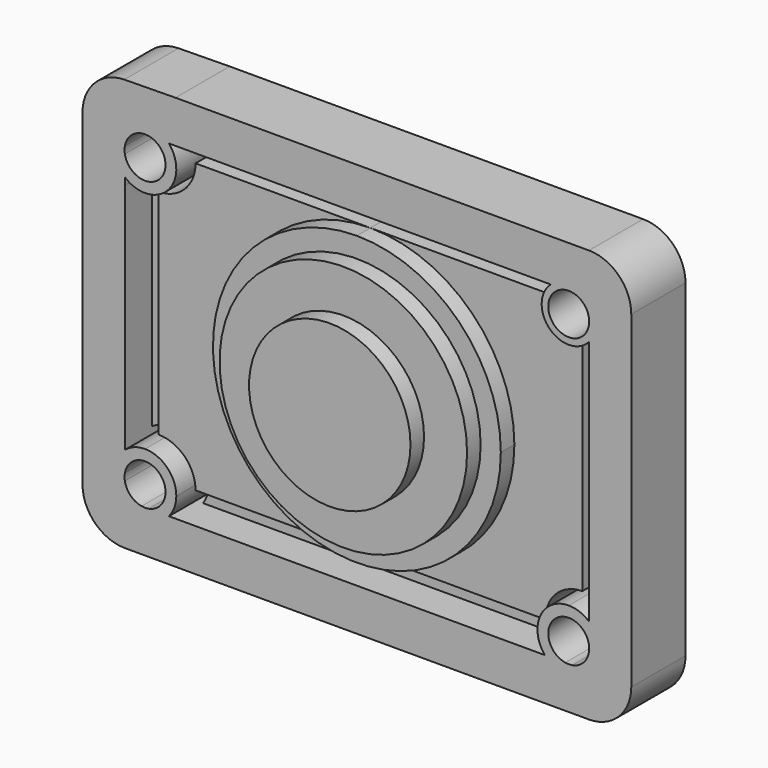
from build123d import *

# Parameters (mm, degrees)
F0_R     = 9.525
F1_DEPTH = 12
F3_DEPTH = 6
F0_R_2   = 14.605
F4_DEPTH = 8
F5_DEPTH = 10
F6_DEPTH = 8
F7_DEPTH = 4


# Not quite as in the source:
# - a feature of the source that left no trace in its solid (it failed there, or was rolled back) is left out


with BuildPart() as f1:
    # F0 (on Front) → F1 (new body)
    with BuildSketch(Plane.XZ):
        with Locations((25, 0.5246010458)):
            Circle(F0_R)
    extrude(amount=F1_DEPTH)


with BuildPart() as f3:
    # F0 (on Front) → F3 (new body)
    with BuildSketch(Plane.XZ):
        with BuildLine():
            ThreePointArc((25, -16.4603989542), (8.015, 0.5246010458), (25, 17.5096010458))
            Line((25, 17.5096010458), (6.92, 17.5096010458))
            Line((6.92, 17.5096010458), (4.365, 17.5096010458))
            ThreePointArc((4.365, 17.5096010458), (3.0865210999, 14.423079946), (0, 13.1446010458))
            Line((0, 13.1446010458), (0, 10.59))
            Line((0, 10.59), (0, 0))
            Line((0, 0), (0, -10.59))
            Line((0, -10.59), (0, -12.0953989542))
            ThreePointArc((0, -12.0953989542), (3.0865210999, -13.3738778543), (4.365, -16.4603989542))
            Line((4.365, -16.4603989542), (25, -16.4603989542))
        make_face()
    extrude(amount=F3_DEPTH)


with BuildPart() as f3b:
    # F0 (on Front) → F3, piece 2 (new body)
    with BuildSketch(Plane.XZ):
        with BuildLine():
            ThreePointArc((25, 17.5096010458), (37.0102086785, 12.5348097243), (41.985, 0.5246010458))
            ThreePointArc((41.985, 0.5246010458), (37.0102086785, -11.4856076326), (25, -16.4603989542))
            Line((25, -16.4603989542), (45.635, -16.4603989542))
            ThreePointArc((45.635, -16.4603989542), (46.9134789001, -13.3738778543), (50, -12.0953989542))
            Line((50, -12.0953989542), (50, 13.8196010458))
            ThreePointArc((50, 13.8196010458), (47.3907759774, 14.9003770233), (46.31, 17.5096010458))
            Line((46.31, 17.5096010458), (25, 17.5096010458))
        make_face()
    extrude(amount=F3_DEPTH)


with BuildPart() as f4:
    # F0 (on Front) → F4 (new body)
    with BuildSketch(Plane.XZ):
        with BuildLine():
            ThreePointArc((25, -16.4603989542), (37.0102086785, -11.4856076326), (41.985, 0.5246010458))
            ThreePointArc((41.985, 0.5246010458), (37.0102086785, 12.5348097243), (25, 17.5096010458))
            ThreePointArc((25, 17.5096010458), (8.015, 0.5246010458), (25, -16.4603989542))
        make_face()
        with Locations((25, 0.5246010458)):
            Circle(F0_R_2, mode=Mode.SUBTRACT)
    extrude(amount=F4_DEPTH)


with BuildPart() as f5:
    # F0 (on Front) → F5 (new body)
    with BuildSketch(Plane.XZ):
        with Locations((25, 0.5246010458)):
            Circle(F0_R_2)
        with Locations((25, 0.5246010458)):
            Circle(F0_R, mode=Mode.SUBTRACT)
    extrude(amount=F5_DEPTH)


with BuildPart() as f6:
    # F0 (on Front) → F6 (new body)
    with BuildSketch(Plane.XZ):
        with BuildLine():
            Line((-7.38, 19.8103227064), (-7.38, 0))
            Line((-7.38, 0), (-7.38, -18.8403989542))
            ThreePointArc((-7.38, -18.8403989542), (-5.9155339059, -22.3759328601), (-2.38, -23.8403989542))
            Line((-2.38, -23.8403989542), (52.38, -23.8403989542))
            ThreePointArc((52.38, -23.8403989542), (55.9155339059, -22.3759328601), (57.38, -18.8403989542))
            Line((57.38, -18.8403989542), (57.38, 0))
            Line((57.38, 0), (57.38, 19.8891702691))
            ThreePointArc((57.38, 19.8891702691), (55.9155339059, 23.4247041751), (52.38, 24.8891702691))
            Line((52.38, 24.8891702691), (3.5934421678, 24.8891702691))
            Line((3.5934421678, 24.8891702691), (-2.4456321687, 24.8098919297))
            ThreePointArc((-2.4456321687, 24.8098919297), (-5.9386627294, 23.3225754847), (-7.38, 19.8103227064))
        make_face()
        with BuildLine():
            ThreePointArc((-0.4096644969, -18.8403989542), (-1.7076628766, -18.1680618307), (-2.38, -16.870063451))
            ThreePointArc((-2.38, -16.870063451), (-2.415, -16.4603989542), (-2.38, -16.0507344573))
            ThreePointArc((-2.38, -16.0507344573), (0.2055784522, -14.0541648633), (2.415, -16.4603989542))
            ThreePointArc((2.415, -16.4603989542), (1.8468303604, -18.0164974793), (0.4096644969, -18.8403989542))
            ThreePointArc((0.4096644969, -18.8403989542), (0, -18.8753989542), (-0.4096644969, -18.8403989542))
        make_face(mode=Mode.SUBTRACT)
        with BuildLine():
            ThreePointArc((52.415, -16.4603989542), (52.4062340909, -16.6659774063), (52.38, -16.870063451))
            ThreePointArc((52.38, -16.870063451), (51.7076628766, -18.1680618307), (50.4096644969, -18.8403989542))
            ThreePointArc((50.4096644969, -18.8403989542), (50, -18.8753989542), (49.5903355031, -18.8403989542))
            ThreePointArc((49.5903355031, -18.8403989542), (48.2923371234, -14.7527360776), (52.38, -16.0507344573))
            ThreePointArc((52.38, -16.0507344573), (52.4062340909, -16.254820502), (52.415, -16.4603989542))
        make_face(mode=Mode.SUBTRACT)
        with BuildLine():
            ThreePointArc((47.8684219461, 19.8896010458), (47.0829452454, 18.8129876189), (46.805, 17.5096010458))
            ThreePointArc((46.805, 17.5096010458), (47.7407938341, 15.25039488), (50, 14.3146010458))
            ThreePointArc((50, 14.3146010458), (51.3033865731, 14.5925462913), (52.38, 15.3780229919))
            Line((52.38, 15.3780229919), (52.38, 14.6897251621))
            Line((52.38, 14.6897251621), (52.38, -12.8013246177))
            Line((52.38, -12.8013246177), (52.38, -13.6405230704))
            ThreePointArc((52.38, -13.6405230704), (51.2670355143, -12.9947502406), (50, -12.7703989542))
            ThreePointArc((50, -12.7703989542), (47.3907759774, -13.8511749316), (46.31, -16.4603989542))
            ThreePointArc((46.31, -16.4603989542), (46.5343512865, -17.7274344684), (47.1801241162, -18.8403989542))
            Line((47.1801241162, -18.8403989542), (46.3409256635, -18.8403989542))
            Line((46.3409256635, -18.8403989542), (3.6590743365, -18.8403989542))
            Line((3.6590743365, -18.8403989542), (2.8198758838, -18.8403989542))
            ThreePointArc((2.8198758838, -18.8403989542), (3.4656487135, -17.7274344684), (3.69, -16.4603989542))
            ThreePointArc((3.69, -16.4603989542), (2.6092240226, -13.8511749316), (0, -12.7703989542))
            ThreePointArc((0, -12.7703989542), (-1.2670355143, -12.9947502406), (-2.38, -13.6405230704))
            Line((-2.38, -13.6405230704), (-2.38, -12.8013246177))
            Line((-2.38, -12.8013246177), (-2.38, 13.8505267094))
            Line((-2.38, 13.8505267094), (-2.3881185942, 14.6965973878))
            ThreePointArc((-2.3881185942, 14.6965973878), (2.6054606766, 14.8966190975), (2.8198758838, 19.8896010458))
            Line((2.8198758838, 19.8896010458), (3.6590743365, 19.8896010458))
            Line((3.6590743365, 19.8896010458), (4.3602697551, 19.8896010458))
            Line((4.3602697551, 19.8896010458), (47.1801241162, 19.8896010458))
            Line((47.1801241162, 19.8896010458), (47.8684219461, 19.8896010458))
        make_face(mode=Mode.SUBTRACT)
        with BuildLine():
            ThreePointArc((2.415, 17.5096010458), (0.2055784522, 15.103366955), (-2.38, 17.099936549))
            ThreePointArc((-2.38, 17.099936549), (-2.415, 17.5096010458), (-2.38, 17.9192655427))
            ThreePointArc((-2.38, 17.9192655427), (-1.7076628766, 19.2172639224), (-0.4096644969, 19.8896010458))
            ThreePointArc((-0.4096644969, 19.8896010458), (0, 19.9246010458), (0.4096644969, 19.8896010458))
            ThreePointArc((0.4096644969, 19.8896010458), (1.8468303604, 19.065699571), (2.415, 17.5096010458))
        make_face(mode=Mode.SUBTRACT)
        with BuildLine():
            ThreePointArc((50, 19.9246010458), (51.7076628766, 19.2172639224), (52.415, 17.5096010458))
            ThreePointArc((52.415, 17.5096010458), (48.3206029126, 15.7741326875), (49.9207139355, 19.9232991877))
            ThreePointArc((49.9207139355, 19.9232991877), (49.9603516241, 19.9242755594), (50, 19.9246010458))
        make_face(mode=Mode.SUBTRACT)
    extrude(amount=F6_DEPTH)


with BuildPart() as f7:
    # F0 (on Front) → F7 (new body)
    with BuildSketch(Plane.XZ):
        with BuildLine():
            Line((45.635, -16.4603989542), (25, -16.4603989542))
            Line((25, -16.4603989542), (4.365, -16.4603989542))
            ThreePointArc((4.365, -16.4603989542), (4.1847989485, -17.7016413804), (3.6590743365, -18.8403989542))
            Line((3.6590743365, -18.8403989542), (46.3409256635, -18.8403989542))
            ThreePointArc((46.3409256635, -18.8403989542), (45.8152010515, -17.7016413804), (45.635, -16.4603989542))
        make_face()
    extrude(amount=F7_DEPTH)


with BuildPart() as f7b:
    # F0 (on Front) → F7, piece 2 (new body)
    with BuildSketch(Plane.XZ):
        with BuildLine():
            ThreePointArc((-2.38, -12.8013246177), (-1.2412424262, -12.2756000056), (0, -12.0953989542))
            Line((0, -12.0953989542), (0, -10.59))
            Line((0, -10.59), (0, 0))
            Line((0, 0), (0, 10.59))
            Line((0, 10.59), (0, 13.1446010458))
            ThreePointArc((0, 13.1446010458), (-1.2412424262, 13.3248020973), (-2.38, 13.8505267094))
            Line((-2.38, 13.8505267094), (-2.38, -12.8013246177))
        make_face()
    extrude(amount=F7_DEPTH)


with BuildPart() as f7c:
    # F0 (on Front) → F7, piece 3 (new body)
    with BuildSketch(Plane.XZ):
        with BuildLine():
            Line((6.92, 17.5096010458), (25, 17.5096010458))
            Line((25, 17.5096010458), (46.31, 17.5096010458))
            ThreePointArc((46.31, 17.5096010458), (46.5343512865, 18.7766365601), (47.1801241162, 19.8896010458))
            Line((47.1801241162, 19.8896010458), (4.3602697551, 19.8896010458))
            Line((4.3602697551, 19.8896010458), (3.6590743365, 19.8896010458))
            ThreePointArc((3.6590743365, 19.8896010458), (4.1847989485, 18.750843472), (4.365, 17.5096010458))
            Line((4.365, 17.5096010458), (6.92, 17.5096010458))
        make_face()
    extrude(amount=F7_DEPTH)


with BuildPart() as f7d:
    # F0 (on Front) → F7, piece 4 (new body)
    with BuildSketch(Plane.XZ):
        with BuildLine():
            ThreePointArc((52.38, 14.6897251621), (51.2670355143, 14.0439523323), (50, 13.8196010458))
            Line((50, 13.8196010458), (50, -12.0953989542))
            ThreePointArc((50, -12.0953989542), (51.2412424262, -12.2756000056), (52.38, -12.8013246177))
            Line((52.38, -12.8013246177), (52.38, 14.6897251621))
        make_face()
    extrude(amount=F7_DEPTH)


solid = Compound([f1.part, f3.part, f3b.part, f4.part, f5.part, f6.part, f7.part, f7b.part, f7c.part, f7d.part])
